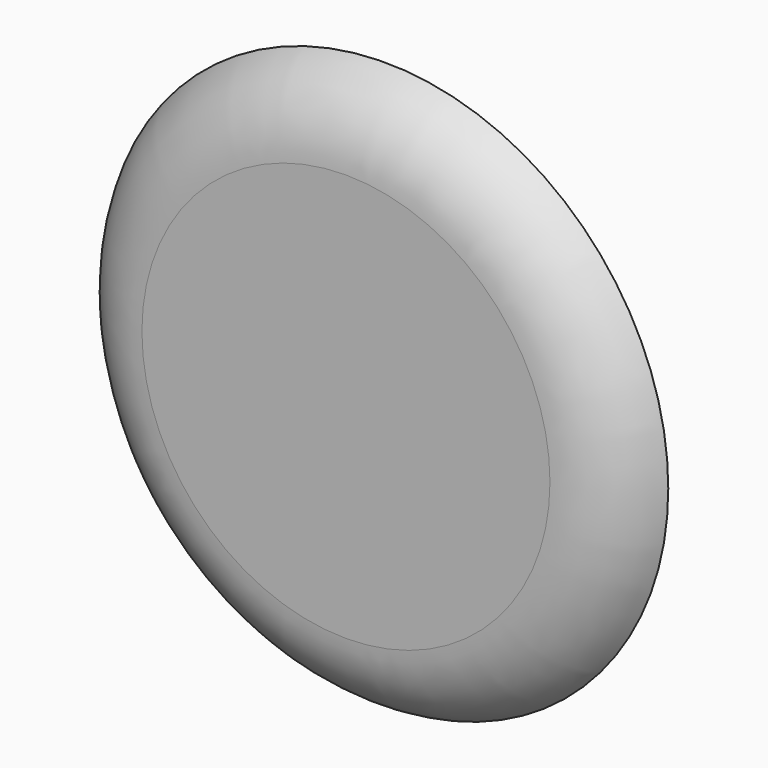
from build123d import *

# Parameters (mm, degrees)
F0_R     = 73.025
F1_DEPTH = 12.7


# Not quite as in the source:
# - a fillet or chamfer that OpenCascade refuses, or shapes differently, is made with other operations: its cross-section is extruded or revolved along the edge and cut away or added


with BuildPart() as f1:
    # F0 (on Front) → F1 (new body)
    with BuildSketch(Plane.XZ):
        Circle(F0_R)
    extrude(amount=F1_DEPTH)

    # F2: fillet of radius 22.6887790592 on 1 edges, made by hand

    # F2_s1 → F2_t2 (revolve, cut)
    with BuildSketch(Plane.XY):
        with BuildLine():
            ThreePointArc((73.025, 0), (64.6564011841, -9.2649724758), (52.6533287847, -12.7))
            Line((52.6533287847, -12.7), (73.025, -12.7))
            Line((73.025, -12.7), (73.025, 0))
        make_face()
    revolve(axis=Axis((0, -12.7, 0), (0, -1, 0)), mode=Mode.SUBTRACT)


solid = f1.part
